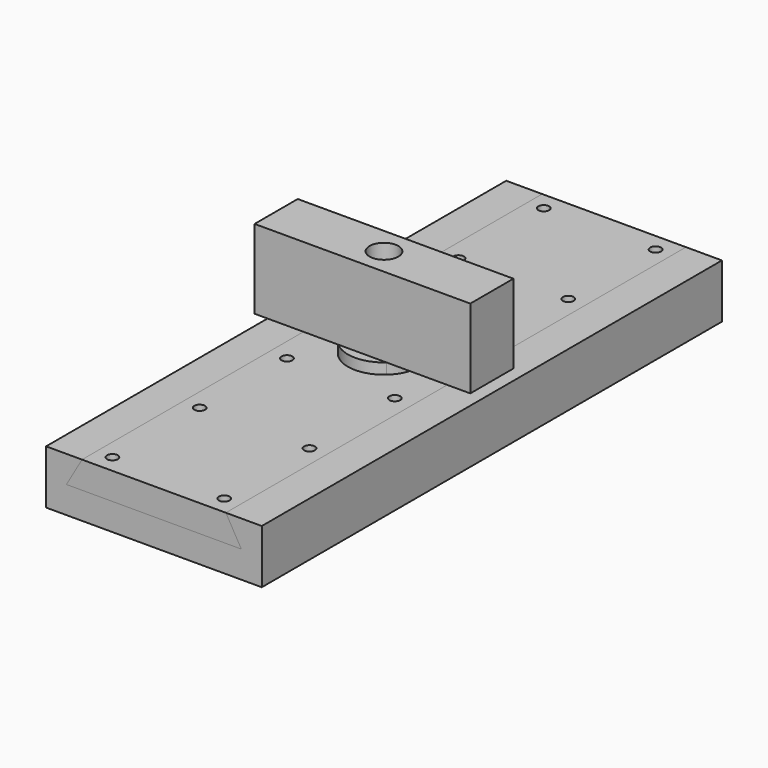
from build123d import *

# Parameters (mm, degrees)
F2_DEPTH      = 80
F2_DEPTH_BACK = 80
F3_DEPTH      = 80
F3_DEPTH_BACK = 80
F4_R          = 4
F5_DEPTH      = 3
F4_W          = 10
F4_H          = 15
F6_DEPTH      = 25
F7_DEPTH      = 3
F8_DEPTH      = 25.001
F8_DEPTH_BACK = 15.001
F9_DEPTH      = 3
F11_DEPTH     = 2
F12_DEPTH     = 15.001
F4_R_2        = 1.5
F13_DEPTH     = 15.001


with BuildPart() as f2:
    # F1 (on Front) → F2 (new body, two sides)
    with BuildSketch(Plane.XZ) as f2_sk:
        Polygon((-30, -7.5), (30, -7.5), (30, 7.5), (20, 7.5), (24.3301270189, 0), (0, 0), (-24.3301270189, 0), (-20, 7.5), (-30, 7.5), align=None)
    extrude(amount=F2_DEPTH)
    extrude(f2_sk.sketch, amount=-F2_DEPTH_BACK)


with BuildPart() as f3:
    # F1 (on Front) → F3 (new body, two sides)
    with BuildSketch(Plane.XZ) as f3_sk:
        Polygon((24.3301270189, 0), (20, 7.5), (-20, 7.5), (-24.3301270189, 0), (0, 0), align=None)
    extrude(amount=F3_DEPTH)
    extrude(f3_sk.sketch, amount=-F3_DEPTH_BACK)

    # F4 (on face) → F5 (cut)
    with BuildSketch(Plane.XY.offset(7.5)):
        with BuildLine():
            ThreePointArc((6.6897309363, -7.5), (9.1715401081, -4.1091789989), (10.05, 0))
            ThreePointArc((10.05, 0), (9.1715401081, 4.1091789989), (6.6897309363, 7.5))
            Line((6.6897309363, 7.5), (-6.6897309363, 7.5))
            ThreePointArc((-6.6897309363, 7.5), (-10.05, 0), (-6.6897309363, -7.5))
            Line((-6.6897309363, -7.5), (6.6897309363, -7.5))
        make_face()
        Circle(F4_R, mode=Mode.SUBTRACT)
        with BuildLine():
            Line((-6.6897309363, 7.5), (6.6897309363, 7.5))
            ThreePointArc((6.6897309363, 7.5), (0, 10.05), (-6.6897309363, 7.5))
        make_face()
        with BuildLine():
            ThreePointArc((-6.6897309363, -7.5), (0, -10.05), (6.6897309363, -7.5))
            Line((6.6897309363, -7.5), (-6.6897309363, -7.5))
        make_face()
    extrude(amount=-F5_DEPTH, mode=Mode.SUBTRACT)

    # F10 (on face) → F11 (cut)
    with BuildSketch(Plane(origin=(0, 0, 0), x_dir=(1, 0, 0), z_dir=(0, 0, -1))):
        Polygon((6.9282032303, 0), (3.4641016151, 6), (-3.4641016151, 6), (-6.9282032303, 0), (-3.4641016151, -6), (3.4641016151, -6), align=None)
    extrude(amount=-F11_DEPTH, mode=Mode.SUBTRACT)

    # F4 (on face) → F12 (cut, through all)
    with BuildSketch(Plane.XY.offset(7.5)):
        Circle(F4_R)
    extrude(amount=-F12_DEPTH, mode=Mode.SUBTRACT)


with BuildPart() as f6:
    # F4 (on face) → F6 (new body)
    with BuildSketch(Plane.XY.offset(7.5)):
        with Locations((-25, 0)):
            Rectangle(F4_W, F4_H)
        with BuildLine():
            ThreePointArc((-6.6897309363, -7.5), (-10.05, 0), (-6.6897309363, 7.5))
            Line((-6.6897309363, 7.5), (-20, 7.5))
            Line((-20, 7.5), (-20, -7.5))
            Line((-20, -7.5), (-6.6897309363, -7.5))
        make_face()
        with BuildLine():
            Line((-6.6897309363, 7.5), (6.6897309363, 7.5))
            ThreePointArc((6.6897309363, 7.5), (0, 10.05), (-6.6897309363, 7.5))
        make_face()
        with BuildLine():
            ThreePointArc((-6.6897309363, -7.5), (0, -10.05), (6.6897309363, -7.5))
            Line((6.6897309363, -7.5), (-6.6897309363, -7.5))
        make_face()
        with BuildLine():
            ThreePointArc((6.6897309363, 7.5), (9.1715401081, 4.1091789989), (10.05, 0))
            ThreePointArc((10.05, 0), (9.1715401081, -4.1091789989), (6.6897309363, -7.5))
            Line((6.6897309363, -7.5), (20, -7.5))
            Line((20, -7.5), (20, 7.5))
            Line((20, 7.5), (6.6897309363, 7.5))
        make_face()
        with BuildLine():
            ThreePointArc((6.6897309363, -7.5), (9.1715401081, -4.1091789989), (10.05, 0))
            ThreePointArc((10.05, 0), (9.1715401081, 4.1091789989), (6.6897309363, 7.5))
            Line((6.6897309363, 7.5), (-6.6897309363, 7.5))
            ThreePointArc((-6.6897309363, 7.5), (-10.05, 0), (-6.6897309363, -7.5))
            Line((-6.6897309363, -7.5), (6.6897309363, -7.5))
        make_face()
        Circle(F4_R, mode=Mode.SUBTRACT)
        with Locations((25, 0)):
            Rectangle(F4_W, F4_H)
    extrude(amount=F6_DEPTH)

    # F4 (on face) → F7 (cut)
    with BuildSketch(Plane.XY.offset(7.5)):
        with Locations((25, 0)):
            Rectangle(F4_W, F4_H)
        with BuildLine():
            ThreePointArc((6.6897309363, 7.5), (9.1715401081, 4.1091789989), (10.05, 0))
            ThreePointArc((10.05, 0), (9.1715401081, -4.1091789989), (6.6897309363, -7.5))
            Line((6.6897309363, -7.5), (20, -7.5))
            Line((20, -7.5), (20, 7.5))
            Line((20, 7.5), (6.6897309363, 7.5))
        make_face()
        with BuildLine():
            ThreePointArc((-6.6897309363, -7.5), (-10.05, 0), (-6.6897309363, 7.5))
            Line((-6.6897309363, 7.5), (-20, 7.5))
            Line((-20, 7.5), (-20, -7.5))
            Line((-20, -7.5), (-6.6897309363, -7.5))
        make_face()
        with Locations((-25, 0)):
            Rectangle(F4_W, F4_H)
    extrude(amount=F7_DEPTH, mode=Mode.SUBTRACT)

    # F4 (on face) → F8 (cut, two sides)
    with BuildSketch(Plane.XY.offset(7.5)) as f8_sk:
        Circle(F4_R)
        with BuildLine():
            Line((-6.6897309363, 7.5), (6.6897309363, 7.5))
            ThreePointArc((6.6897309363, 7.5), (0, 10.05), (-6.6897309363, 7.5))
        make_face()
        with BuildLine():
            ThreePointArc((-6.6897309363, -7.5), (0, -10.05), (6.6897309363, -7.5))
            Line((6.6897309363, -7.5), (-6.6897309363, -7.5))
        make_face()
    extrude(amount=F8_DEPTH, mode=Mode.SUBTRACT)
    extrude(f8_sk.sketch, amount=-F8_DEPTH_BACK, mode=Mode.SUBTRACT)

    # F4 (on face) → F9 (join)
    with BuildSketch(Plane.XY.offset(7.5)):
        with BuildLine():
            Line((-6.6897309363, 7.5), (6.6897309363, 7.5))
            ThreePointArc((6.6897309363, 7.5), (0, 10.05), (-6.6897309363, 7.5))
        make_face()
        with BuildLine():
            ThreePointArc((-6.6897309363, -7.5), (0, -10.05), (6.6897309363, -7.5))
            Line((6.6897309363, -7.5), (-6.6897309363, -7.5))
        make_face()
    extrude(amount=F9_DEPTH)


with BuildPart() as f13_tool:
    # F4 (on face) → F13 (new body, through all)
    with BuildSketch(Plane.XY.offset(7.5)):
        with Locations((15, 15)):
            Circle(F4_R_2)
        with Locations((15.2727160037, 44.9987604074)):
            Circle(F4_R_2)
        with Locations((-15.2727160037, 44.9987604074)):
            Circle(F4_R_2)
        with Locations((-15, 15)):
            Circle(F4_R_2)
        with Locations((-15, -15)):
            Circle(F4_R_2)
        with Locations((15, -15)):
            Circle(F4_R_2)
        with Locations((15.2727160037, -44.9987604074)):
            Circle(F4_R_2)
        with Locations((-15.2727160037, -44.9987604074)):
            Circle(F4_R_2)
        with Locations((-15.5454320074, -74.9975208148)):
            Circle(F4_R_2)
        with Locations((15.5454320074, -74.9975208148)):
            Circle(F4_R_2)
        with Locations((15.5454320074, 74.9975208148)):
            Circle(F4_R_2)
        with Locations((-15.5454320074, 74.9975208148)):
            Circle(F4_R_2)
    extrude(amount=-F13_DEPTH)


with BuildPart() as f2_1:
    add(f2.part)

    # F13: cut by f13_tool
    add(f13_tool.part, mode=Mode.SUBTRACT)


with BuildPart() as f3_1:
    add(f3.part)

    # F13: cut by f13_tool
    add(f13_tool.part, mode=Mode.SUBTRACT)


solid = Compound([f6.part, f2_1.part, f3_1.part])
